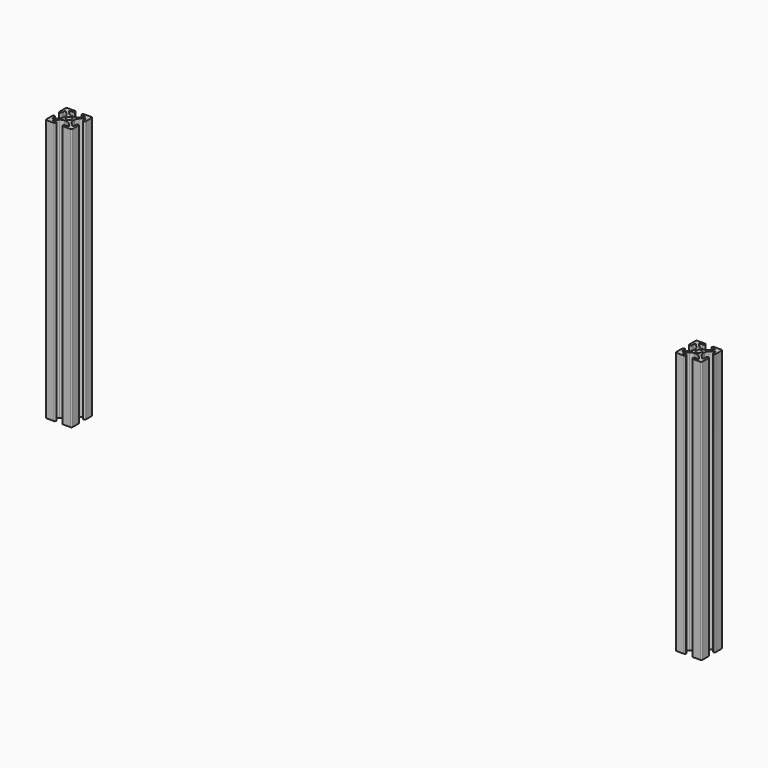
from build123d import *

# Parameters (mm, degrees)
F0_R     = 2.6035
F1_DEPTH = 254
F2_R     = 1.18109
F3_R     = 5.08
F4_R     = 0.762
F5_R     = 1.27


# Not quite as in the source:
# - a fillet or chamfer is up to 0.001 mm smaller than in the source, because OpenCascade refuses the exact size


with BuildPart() as f1:
    # F0 (on Top) → F1 (new body)
    with BuildSketch(Plane.XY):
        Polygon((12.7, 3.2385), (12.7, 12.7), (3.2385, 12.7), (3.2385, 10.3378), (8.7752354349, 10.3378), (2.9459354349, 4.5085), (-2.9459354349, 4.5085), (-8.7752354349, 10.3378), (-3.2385, 10.3378), (-3.2385, 12.7), (-12.7, 12.7), (-12.7, 3.2385), (-10.3378, 3.2385), (-10.3378, 8.7752354349), (-4.5085, 2.9459354349), (-4.5085, -2.9459354349), (-10.3378, -8.7752354349), (-10.3378, -3.2385), (-12.7, -3.2385), (-12.7, -12.7), (-3.2385, -12.7), (-3.2385, -10.3378), (-8.7752354349, -10.3378), (-2.9459354349, -4.5085), (2.9459354349, -4.5085), (8.7752354349, -10.3378), (3.2385, -10.3378), (3.2385, -12.7), (12.7, -12.7), (12.7, -3.2385), (10.3378, -3.2385), (10.3378, -8.7752354349), (4.5085, -2.9459354349), (4.5085, 2.9459354349), (10.3378, 8.7752354349), (10.3378, 3.2385), align=None)
        Circle(F0_R, mode=Mode.SUBTRACT)
    extrude(amount=F1_DEPTH)

    # F2 (radius 1.1811 in the source; OpenCascade refuses exactly that, so slightly less here)
    f2_edges = [f1.edges().sort_by_distance(p)[0] for p in [
        (3.2385, 12.7, 127),
        (3.2385, 10.3378, 127),
        (-3.2385, 12.7, 127),
        (-12.7, 3.2385, 127),
        (-3.2385, 10.3378, 127),
        (-10.3378, 3.2385, 127),
        (12.7, 3.2385, 127),
        (10.3378, 3.2385, 127),
        (12.7, -3.2385, 127),
        (10.3378, -3.2385, 127),
        (3.2385, -10.3378, 127),
        (-3.2385, -10.3378, 127),
        (-10.3378, -3.2385, 127),
        (-12.7, -3.2385, 127),
        (-3.2385, -12.7, 127),
        (3.2385, -12.7, 127),
    ]]
    fillet(f2_edges, radius=F2_R)

    # F3
    f3_edges = [f1.edges().sort_by_distance(p)[0] for p in [
        (2.945935, 4.5085, 127),
        (-2.945935, 4.5085, 127),
        (4.5085, -2.945935, 127),
        (4.5085, 2.945935, 127),
        (2.945935, -4.5085, 127),
        (-2.945935, -4.5085, 127),
        (-4.5085, -2.945935, 127),
        (-4.5085, 2.945935, 127),
    ]]
    fillet(f3_edges, radius=F3_R)

    # F4
    f4_edges = [f1.edges().sort_by_distance(p)[0] for p in [
        (8.775235, 10.3378, 127),
        (-8.775235, 10.3378, 127),
        (-10.3378, 8.775235, 127),
        (-10.3378, -8.775235, 127),
        (-8.775235, -10.3378, 127),
        (8.775235, -10.3378, 127),
        (10.3378, -8.775235, 127),
        (10.3378, 8.775235, 127),
    ]]
    fillet(f4_edges, radius=F4_R)

    # F5
    f5_edges = [f1.edges().sort_by_distance(p)[0] for p in [
        (-12.7, -12.7, 127),
        (12.7, -12.7, 127),
        (12.7, 12.7, 127),
        (-12.7, 12.7, 127),
    ]]
    fillet(f5_edges, radius=F5_R)


with BuildPart() as f6_1:
    # F6: copy of F1
    add(f1.part.moved(Location((609.6, 0, 0))))


solid = Compound([f1.part, f6_1.part])
